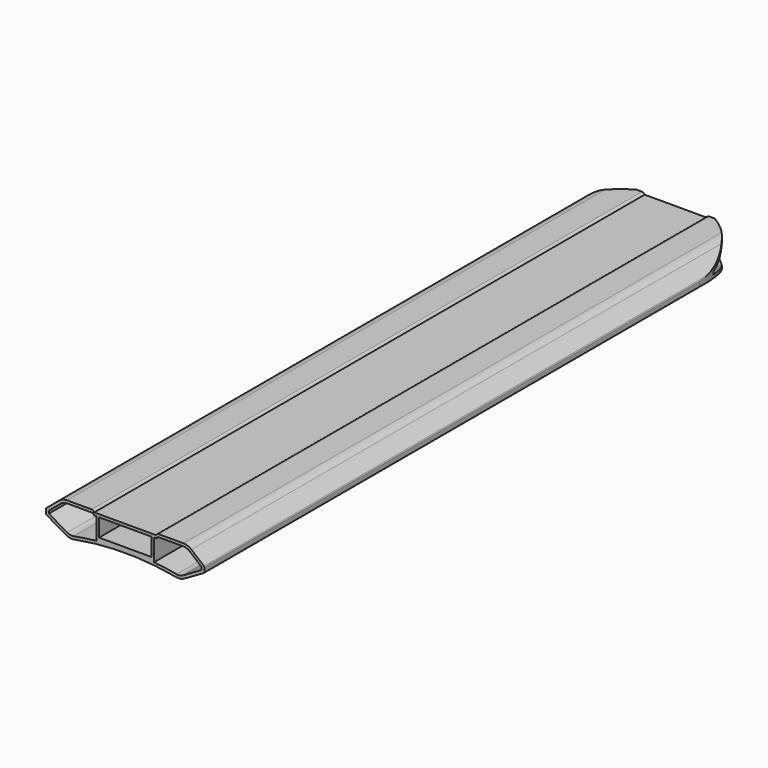
from build123d import *

# Parameters (mm, degrees)
F1_DEPTH       = 250
F2_W           = 38
F2_H           = 13
F3_DEPTH       = 1200
F5_R           = 9
F6_R           = 1
F9_DEPTH       = 500.001
F11_DEPTH      = 23.8214951236
F11_DEPTH_BACK = 526


# Not quite as in the source:
# - an extrude ends at something that could not be found from the text; its depth is read off the source's solid
# - a feature of the source that left no trace in its solid (it failed there, or was rolled back) is left out


with BuildPart() as f1:
    # F0 (on Front) → F1 (new body, symmetric)
    with BuildSketch(Plane.XZ):
        with BuildLine():
            Line((22.5, 62.3204951236), (0, 62.3204951236))
            Line((0, 62.3204951236), (-22.5, 62.3204951236))
            Line((-22.5, 62.3204951236), (-22.5, 63.6204951236))
            Line((-22.5, 63.6204951236), (-45.5824640741, 63.6204951236))
            Line((-45.5824640741, 63.6204951236), (-57.5, 53.6204951236))
            Line((-57.5, 53.6204951236), (-57.5, 49.6204951236))
            Line((-57.5, 49.6204951236), (-40.1794919243, 39.6204951236))
            ThreePointArc((-40.1794919243, 39.6204951236), (0, 43.698039982), (40.1794919243, 39.6204951236))
            Line((40.1794919243, 39.6204951236), (57.5, 49.6204951236))
            Line((57.5, 49.6204951236), (57.5, 53.6204951236))
            Line((57.5, 53.6204951236), (45.5824640741, 63.6204951236))
            Line((45.5824640741, 63.6204951236), (22.5, 63.6204951236))
            Line((22.5, 63.6204951236), (22.5, 62.3204951236))
        make_face()
    extrude(amount=F1_DEPTH, both=True)

    # F2 (on face) → F3 (cut)
    with BuildSketch(Plane.XZ.offset(250)):
        with Locations((0, 53.8204951236)):
            Rectangle(F2_W, F2_H)
    extrude(amount=-F3_DEPTH, mode=Mode.SUBTRACT)

    # F5
    f5_edges = [f1.edges().sort_by_distance(p)[0] for p in [
        (45.582464, 0, 63.620495),
        (40.179492, 0, 39.620495),
        (-40.179492, 0, 39.620495),
        (-45.582464, 0, 63.620495),
    ]]
    fillet(f5_edges, radius=F5_R)

    # F6
    f6_edges = [f1.edges().sort_by_distance(p)[0] for p in [
        (-57.5, 0, 53.620495),
        (-57.5, 0, 49.620495),
        (57.5, 0, 53.620495),
        (57.5, 0, 49.620495),
    ]]
    fillet(f6_edges, radius=F6_R)


with BuildPart() as f1_1:
    # F7: moved
    add(f1.part.moved(Location((0, 0, -39.8))))

    # F8 (on face) → F9 (cut, through all)
    with BuildSketch(Plane.XZ.offset(250)):
        with BuildLine():
            ThreePointArc((22.5, 22.5204951236), (23.2333239744, 23.4636627961), (24.3734993995, 23.8204951236))
            Line((24.3734993995, 23.8204951236), (22.5, 23.8204951236))
            Line((22.5, 23.8204951236), (22.5, 22.5204951236))
        make_face()
        with BuildLine():
            ThreePointArc((-24.3734993995, 23.8204951236), (-23.2333239744, 23.4636627961), (-22.5, 22.5204951236))
            Line((-22.5, 22.5204951236), (-22.5, 23.8204951236))
            Line((-22.5, 23.8204951236), (-24.3734993995, 23.8204951236))
        make_face()
        with BuildLine():
            ThreePointArc((-42.1022690923, 3.2400121158), (-39.7790673433, 2.4018170628), (-37.3093701274, 2.4226251111))
            ThreePointArc((-37.3093701274, 2.4226251111), (-29.1789785809, 3.779472859), (-21, 4.8034903809))
            Line((-21, 4.8034903809), (-21, 20.5204952508))
            Line((-21, 20.5204952508), (-22.5, 20.5204952508))
            ThreePointArc((-22.5, 20.5204952508), (-23.2333240107, 21.4636628361), (-24.3734993995, 21.8204951236))
            Line((-24.3734993995, 21.8204951236), (-42.3067319657, 21.8204951236))
            ThreePointArc((-42.3067319657, 21.8204951236), (-44.7008729689, 21.3983434691), (-46.8062452335, 20.1828062254))
            Line((-46.8062452335, 20.1828062254), (-55.5, 12.8878798072))
            Line((-55.5, 12.8878798072), (-55.5, 10.9751956619))
            Line((-55.5, 10.9751956619), (-42.1022690923, 3.2400121158))
        make_face()
        with BuildLine():
            ThreePointArc((24.3734993995, 21.8204951236), (23.2333240107, 21.4636628361), (22.5, 20.5204952508))
            Line((22.5, 20.5204952508), (21, 20.5204952508))
            Line((21, 20.5204952508), (21, 4.8034903809))
            ThreePointArc((21, 4.8034903809), (29.1789785809, 3.779472859), (37.3093701274, 2.4226251111))
            ThreePointArc((37.3093701274, 2.4226251111), (39.7790673433, 2.4018170628), (42.1022690923, 3.2400121158))
            Line((42.1022690923, 3.2400121158), (55.5, 10.9751956619))
            Line((55.5, 10.9751956619), (55.5, 12.8878798072))
            Line((55.5, 12.8878798072), (46.8062452335, 20.1828062254))
            ThreePointArc((46.8062452335, 20.1828062254), (44.7008729689, 21.3983434691), (42.3067319657, 21.8204951236))
            Line((42.3067319657, 21.8204951236), (24.3734993995, 21.8204951236))
        make_face()
    extrude(amount=-F9_DEPTH, mode=Mode.SUBTRACT)

    # F10 (on Top) → F11 (cut, two sides)
    with BuildSketch(Plane.XY) as f11_sk:
        with BuildLine():
            ThreePointArc((-57.5, 200), (0, 257.5), (57.5, 200))
            Line((57.5, 200), (57.5, 280))
            Line((57.5, 280), (-57.5, 280))
            Line((-57.5, 280), (-57.5, 200))
        make_face()
    extrude(amount=F11_DEPTH, mode=Mode.SUBTRACT)
    extrude(f11_sk.sketch, amount=-F11_DEPTH_BACK, mode=Mode.SUBTRACT)


solid = f1_1.part
